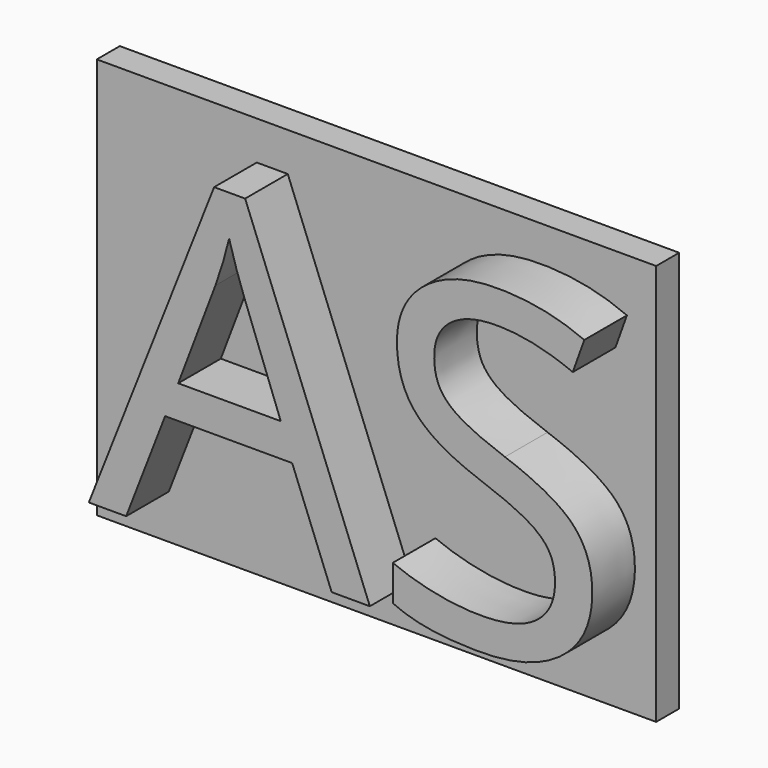
from build123d import *

# Parameters (mm, degrees)
F0_TEXT_SIZE = 105.8333333333
F1_DEPTH     = 12.7
F2_W         = 133.3167850971
F2_H         = 95.6533029675
F3_DEPTH     = 6.858


# Not quite as in the source:
# - Text() gives the source's letters only with a copy of the font that has no kerning and outlines rounded to 1/6400 em; it was checked with that copy


with BuildPart() as f1:
    # F0 (on Front) → F1 (new body)
    with BuildSketch(Plane.XZ):
        with Locations((-44.7472346874, -44.2608505157)):
            Text('AS', F0_TEXT_SIZE, font='Open Sans', text_align=(TextAlign.LEFT, TextAlign.BOTTOM))
    extrude(amount=F1_DEPTH)

    # F2 (on Front) → F3 (join)
    with BuildSketch(Plane.XZ):
        with Locations((13.650521636, -6.9747194648)):
            Rectangle(F2_W, F2_H)
    extrude(amount=-F3_DEPTH)


solid = f1.part
